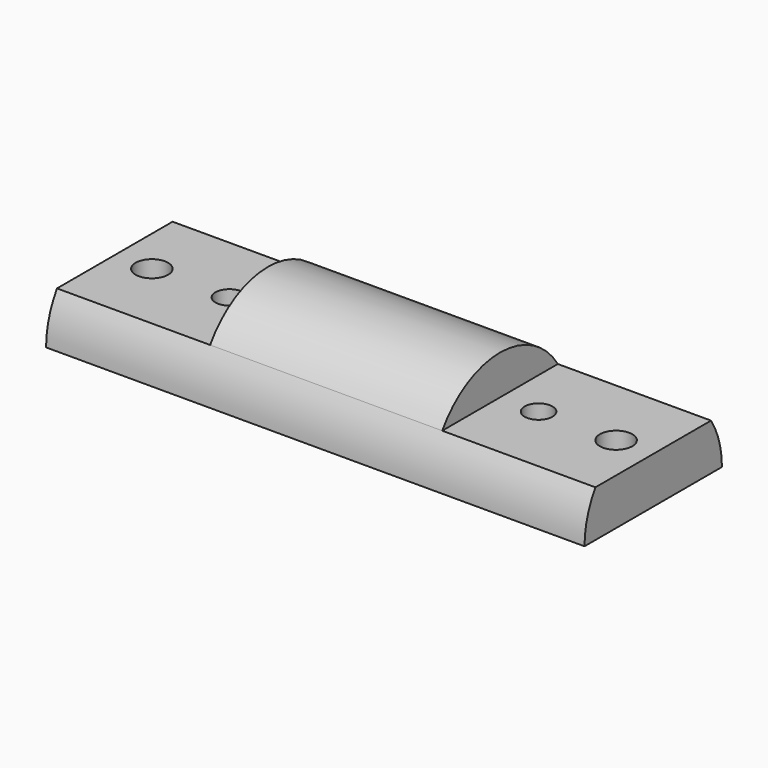
from build123d import *

# Parameters (mm, degrees)
F0_W     = 38
F0_H     = 18.5
F0_R     = 1.5
F0_W_2   = 10
F0_R_2   = 1.75
F1_DEPTH = 5
F2_W     = 25
F2_H     = 18.5
F3_DEPTH = 9.25
F5_DEPTH = 58.001


with BuildPart() as f1:
    # F0 (on Top) → F1 (new body)
    with BuildSketch(Plane.XY):
        Rectangle(F0_W, F0_H)
        with Locations((-16.65, 0)):
            Circle(F0_R, mode=Mode.SUBTRACT)
        with Locations((16.65, 0)):
            Circle(F0_R, mode=Mode.SUBTRACT)
        with Locations((24, 0)):
            Rectangle(F0_W_2, F0_H)
        with Locations((25, 0)):
            Circle(F0_R_2, mode=Mode.SUBTRACT)
        with Locations((-24, 0)):
            Rectangle(F0_W_2, F0_H)
        with Locations((-25, 0)):
            Circle(F0_R_2, mode=Mode.SUBTRACT)
    extrude(amount=F1_DEPTH)

    # F2 (on face) → F3 (join)
    with BuildSketch(Plane.XY.offset(5)):
        Rectangle(F2_W, F2_H)
    extrude(amount=F3_DEPTH)

    # F4 (on face) → F5 (cut, through all)
    with BuildSketch(Plane(origin=(-29, 0, 0), x_dir=(0, -1, 0), z_dir=(-1, 0, 0))):
        with BuildLine():
            Line((9.25, 5), (9.25, 0))
            Line((9.25, 0), (9.75, 0))
            Line((9.75, 0), (9.75, 19))
            Line((9.75, 19), (-9.25, 19))
            Line((-9.25, 19), (-9.25, 5))
            Line((-9.25, 5), (-7.7821912081, 5))
            ThreePointArc((-7.7821912081, 5), (0, 9.25), (7.7821912081, 5))
            Line((7.7821912081, 5), (9.25, 5))
        make_face()
        with BuildLine():
            ThreePointArc((7.7821912081, 5), (8.8754653026, 2.6054972006), (9.25, 0))
            Line((9.25, 0), (9.25, 5))
            Line((9.25, 5), (7.7821912081, 5))
        make_face()
        with BuildLine():
            Line((-9.25, 5), (-9.25, 0))
            ThreePointArc((-9.25, 0), (-8.8754653026, 2.6054972006), (-7.7821912081, 5))
            Line((-7.7821912081, 5), (-9.25, 5))
        make_face()
    extrude(amount=-F5_DEPTH, mode=Mode.SUBTRACT)


solid = f1.part
